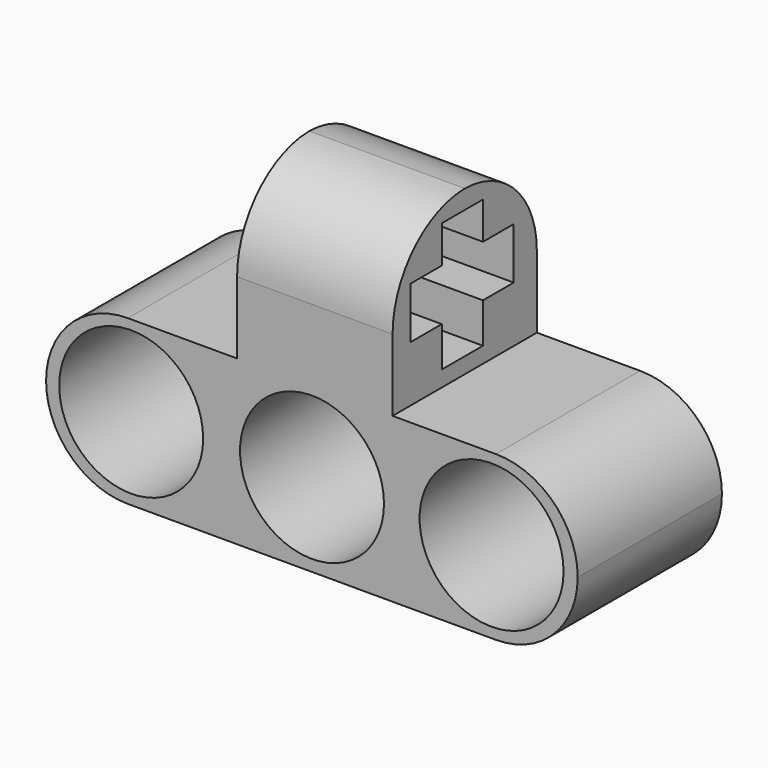
from build123d import *

# Parameters (mm, degrees)
F0_W        = 20.6375
F0_H        = 7
F1_DEPTH    = 6.35
F2_R        = 2.794
F3_DEPTH    = 8
F4_R        = 3.17499
F5_W        = 6.0368906707
F5_H        = 7
F6_DEPTH    = 6.35
F7_T1_DEPTH = 23.8168906707
F8_W        = 2
F8_H        = 5
F9_DEPTH    = 6.35
F10_W       = 1.5076477192
F10_H       = 2
F10_W_2     = 1.4923522808
F10_W_3     = 2
F10_H_2     = 1.5520717202
F11_DEPTH   = 6.35


# Not quite as in the source:
# - a fillet or chamfer that OpenCascade refuses, or shapes differently, is made with other operations: its cross-section is extruded or revolved along the edge and cut away or added
# - a fillet or chamfer is up to 0.001 mm smaller than in the source, because OpenCascade refuses the exact size


with BuildPart() as f1:
    # F0 (on Top) → F1 (new body)
    with BuildSketch(Plane.XY):
        with Locations((1.5829298645, -12.5110630834)):
            Rectangle(F0_W, F0_H)
    extrude(amount=F1_DEPTH)

    # F2 (on face) → F3 (cut)
    with BuildSketch(Plane.XZ.offset(16.0110630834)):
        with Locations((-5.4325845507, 3.1855095279)):
            Circle(F2_R)
        with Locations((1.5883980845, 3.2361580911)):
            Circle(F2_R)
        with Locations((8.5595190756, 3.1868351264)):
            Circle(F2_R)
    extrude(amount=-F3_DEPTH, mode=Mode.SUBTRACT)

    # F4 (radius 3.175 in the source; OpenCascade refuses exactly that, so slightly less here)
    f4_edges = [f1.edges().sort_by_distance(p)[0] for p in [
        (11.90168, -12.511063, 6.35),
        (11.90168, -12.511063, 0),
        (-8.73582, -12.511063, 6.35),
        (-8.73582, -12.511063, 0),
    ]]
    fillet(f4_edges, radius=F4_R)

    # F5 (on face) → F6 (join)
    with BuildSketch(Plane.XY.offset(6.35)):
        with Locations((1.6981104854, -12.5110630834)):
            Rectangle(F5_W, F5_H)
    extrude(amount=F6_DEPTH)

    # F7: fillet of radius 3.556 on 2 edges, made by hand

    # F7_s2 → F7_t1 (cut)
    with BuildSketch(Plane.YZ.offset(-10.2103348499)):
        with BuildLine():
            ThreePointArc((-16.0110630834, 9.144), (-14.9695347973, 11.6584717139), (-12.4550630834, 12.7))
            Line((-12.4550630834, 12.7), (-16.0110630834, 12.7))
            Line((-16.0110630834, 12.7), (-16.0110630834, 9.144))
        make_face()
        with BuildLine():
            ThreePointArc((-9.0110630834, 9.144), (-10.0525913695, 11.6584717139), (-12.5670630834, 12.7))
            Line((-12.5670630834, 12.7), (-9.0110630834, 12.7))
            Line((-9.0110630834, 12.7), (-9.0110630834, 9.144))
        make_face()
    extrude(amount=F7_T1_DEPTH, mode=Mode.SUBTRACT)

    # F8 (on face) → F9 (cut)
    with BuildSketch(Plane(origin=(-1.3203348499, 0, 0), x_dir=(0, -1, 0), z_dir=(-1, 0, 0))):
        with Locations((12.6245897673, 9.4653457722)):
            Rectangle(F8_W, F8_H)
    extrude(amount=-F9_DEPTH, mode=Mode.SUBTRACT)

    # F10 (on face) → F11 (cut)
    with BuildSketch(Plane.YZ.offset(4.7165558208)):
        with Locations((-14.3784136269, 9.5174174924)):
            Rectangle(F10_W, F10_H)
        with Locations((-10.8784136269, 9.5174174924)):
            Rectangle(F10_W_2, F10_H)
        with Locations((-12.6245897673, 7.7413816323)):
            Rectangle(F10_W_3, F10_H_2)
    extrude(amount=-F11_DEPTH, mode=Mode.SUBTRACT)


solid = f1.part
